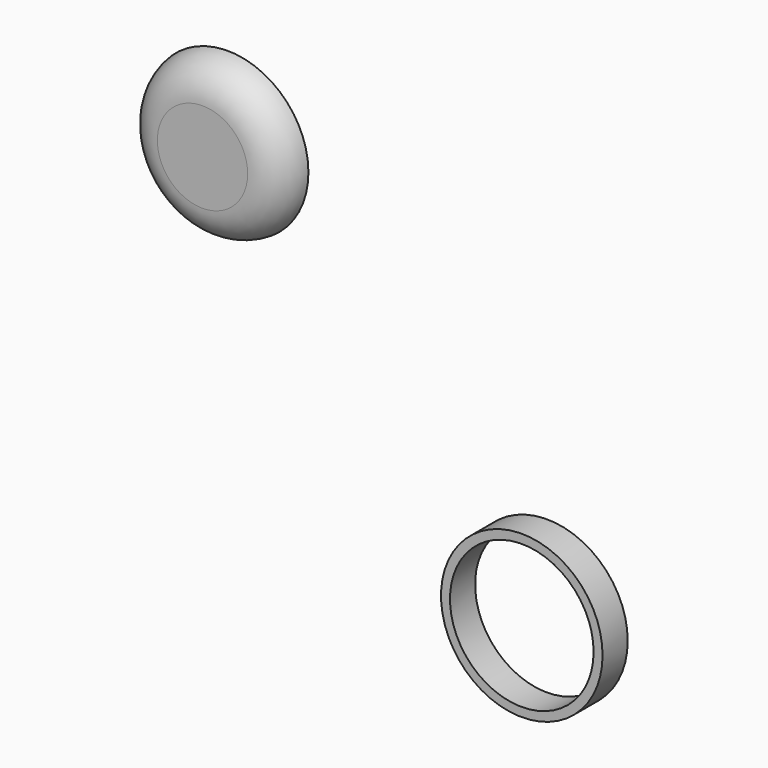
from build123d import *

# Parameters (mm, degrees)
F0_R     = 11.43
F0_R_2   = 10.16
F1_DEPTH = 4.445
F2_R     = 11.43
F3_DEPTH = 4.445


# Not quite as in the source:
# - a fillet or chamfer that OpenCascade refuses, or shapes differently, is made with other operations: its cross-section is extruded or revolved along the edge and cut away or added


with BuildPart() as f1:
    # F0 (on Front) → F1 (new body)
    with BuildSketch(Plane.XZ):
        Circle(F0_R)
        Circle(F0_R_2, mode=Mode.SUBTRACT)
    extrude(amount=F1_DEPTH)


with BuildPart() as f3:
    # F2 (on Front) → F3 (new body)
    with BuildSketch(Plane.XZ):
        with Locations((-45.1791472733, 43.6647646129)):
            Circle(F2_R)
    extrude(amount=F3_DEPTH)

    # F4: fillet of radius 5.08 on 1 edges, made by hand

    # F4_s1 → F4_t2 (revolve, cut)
    with BuildSketch(Plane.XY.offset(43.6647646129)):
        with BuildLine():
            ThreePointArc((-33.7491472733, 0), (-35.4291993558, -3.175), (-38.7893035209, -4.445))
            Line((-38.7893035209, -4.445), (-33.7491472733, -4.445))
            Line((-33.7491472733, -4.445), (-33.7491472733, 0))
        make_face()
    revolve(axis=Axis((-45.1791472733, -4.445, 43.6647646129), (0, -1, 0)), mode=Mode.SUBTRACT)


solid = Compound([f1.part, f3.part])
